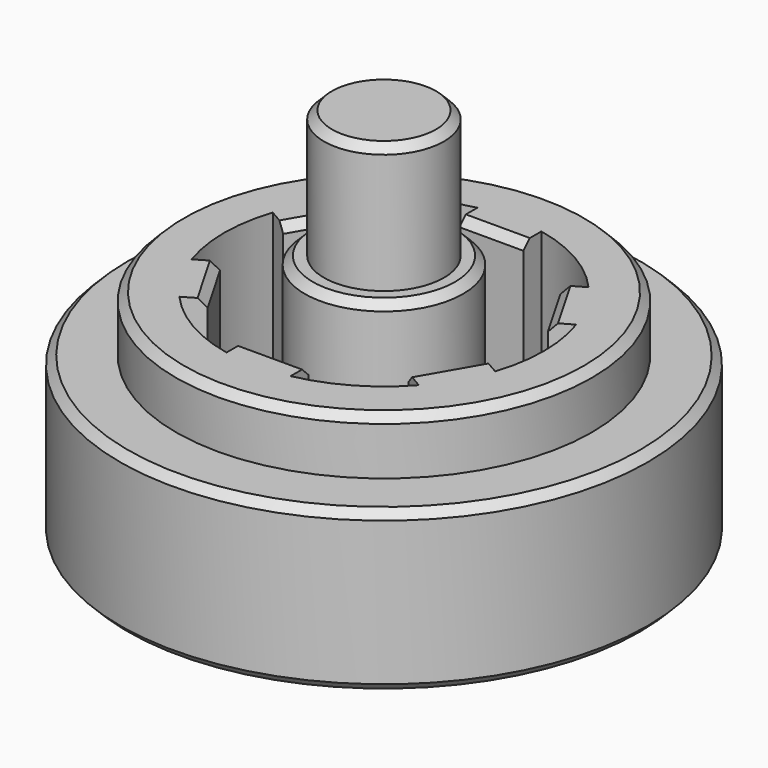
from build123d import *

# Parameters (mm, degrees)
F0_R      = 16.5
F1_DEPTH  = 10
F2_R      = 13
F3_DEPTH  = 10.5
F4_SIZE   = 0.5
F5_R      = 4.95
F6_DEPTH  = 12.5
F7_SIZE   = 0.5
F8_R      = 3.75
F9_DEPTH  = 8
F10_SIZE  = 0.5
F11_R     = 16.5
F11_R_2   = 13
F12_DEPTH = 7
F13_R     = 25
F14_DEPTH = 7
F15_SIZE  = 0.5


with BuildPart() as f1:
    # F0 (on Top) → F1 (new body)
    with BuildSketch(Plane.XY):
        Circle(F0_R)
    extrude(amount=F1_DEPTH)

    # F2 (on face) → F3 (join)
    with BuildSketch(Plane.XY.offset(10)):
        Circle(F2_R)
        with BuildLine():
            ThreePointArc((-7.4852813742, 6.6310302931), (-5, 8.6602540378), (-2, 9.7979589711))
            Line((-2, 9.7979589711), (-2, 8.4))
            Line((-2, 8.4), (2, 8.4))
            Line((2, 8.4), (2, 9.7979589711))
            ThreePointArc((2, 9.7979589711), (5, 8.6602540378), (7.4852813742, 6.6310302931))
            Line((7.4852813742, 6.6310302931), (6.2746133918, 5.9320508076))
            Line((6.2746133918, 5.9320508076), (8.2746133918, 2.4679491924))
            Line((8.2746133918, 2.4679491924), (9.4852813742, 3.166928678))
            ThreePointArc((9.4852813742, 3.166928678), (10, 0), (9.4852813742, -3.166928678))
            Line((9.4852813742, -3.166928678), (8.2746133918, -2.4679491924))
            Line((8.2746133918, -2.4679491924), (6.2746133918, -5.9320508076))
            Line((6.2746133918, -5.9320508076), (7.4852813742, -6.6310302931))
            ThreePointArc((7.4852813742, -6.6310302931), (5, -8.6602540378), (2, -9.7979589711))
            Line((2, -9.7979589711), (2, -8.4))
            Line((2, -8.4), (-2, -8.4))
            Line((-2, -8.4), (-2, -9.7979589711))
            ThreePointArc((-2, -9.7979589711), (-5, -8.6602540378), (-7.4852813742, -6.6310302931))
            Line((-7.4852813742, -6.6310302931), (-6.2746133918, -5.9320508076))
            Line((-6.2746133918, -5.9320508076), (-8.2746133918, -2.4679491924))
            Line((-8.2746133918, -2.4679491924), (-9.4852813742, -3.166928678))
            ThreePointArc((-9.4852813742, -3.166928678), (-10, 0), (-9.4852813742, 3.166928678))
            Line((-9.4852813742, 3.166928678), (-8.2746133918, 2.4679491924))
            Line((-8.2746133918, 2.4679491924), (-6.2746133918, 5.9320508076))
            Line((-6.2746133918, 5.9320508076), (-7.4852813742, 6.6310302931))
        make_face(mode=Mode.SUBTRACT)
    extrude(amount=F3_DEPTH)

    # F4
    f4_edges = [f1.edges().sort_by_distance(p)[0] for p in [
        (0, 8.4, 20.5),
        (-7.274613, 4.2, 20.5),
        (-7.274613, -4.2, 20.5),
        (0, -8.4, 20.5),
        (7.274613, -4.2, 20.5),
        (7.274613, 4.2, 20.5),
    ]]
    chamfer(f4_edges, length=F4_SIZE)

    # F5 (on face) → F6 (join)
    with BuildSketch(Plane.XY.offset(10)):
        Circle(F5_R)
    extrude(amount=F6_DEPTH)

    # F7
    f7_edges = [f1.edges().sort_by_distance(p)[0] for p in [
        (-4.95, 0, 22.5),
    ]]
    chamfer(f7_edges, length=F7_SIZE)

    # F8 (on face) → F9 (join)
    with BuildSketch(Plane.XY.offset(22.5)):
        Circle(F8_R)
    extrude(amount=F9_DEPTH)

    # F10
    f10_edges = [f1.edges().sort_by_distance(p)[0] for p in [
        (-3.75, 0, 30.5),
    ]]
    chamfer(f10_edges, length=F10_SIZE)

    # F11 (on face) → F12 (join)
    with BuildSketch(Plane.XY.offset(10)):
        Circle(F11_R)
        Circle(F11_R_2, mode=Mode.SUBTRACT)
    extrude(amount=F12_DEPTH)

    # F13 (on face) → F14 (cut)
    with BuildSketch(Plane(origin=(0, 0, 0), x_dir=(1, 0, 0), z_dir=(0, 0, -1))):
        Circle(F13_R)
    extrude(amount=-F14_DEPTH, mode=Mode.SUBTRACT)

    # F15
    f15_edges = [f1.edges().sort_by_distance(p)[0] for p in [
        (-13, 0, 20.5),
        (-16.5, 0, 17),
        (-16.5, 0, 7),
    ]]
    chamfer(f15_edges, length=F15_SIZE)


solid = f1.part
